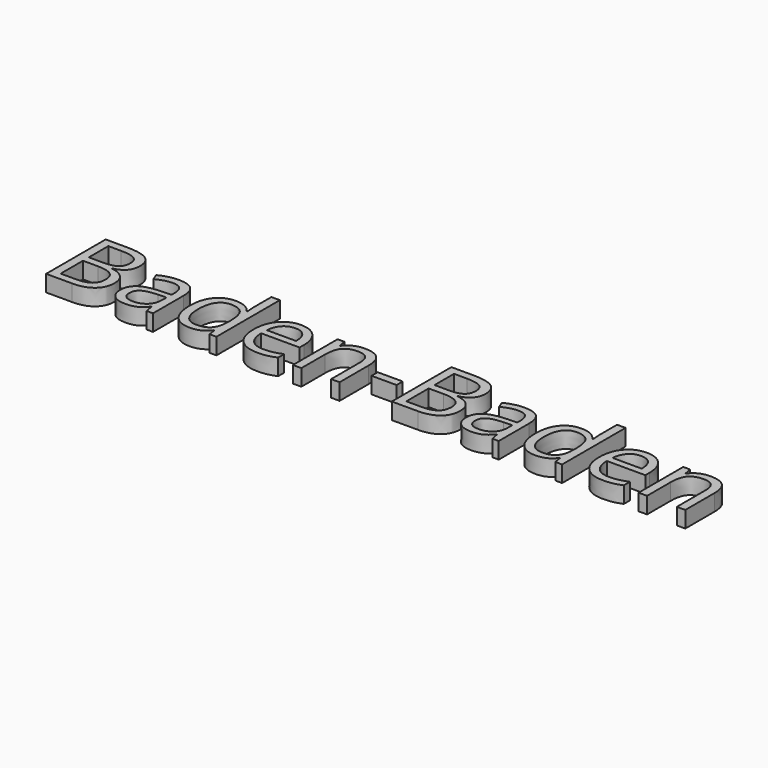
from build123d import *

# Parameters (mm, degrees)
F0_TEXT_SIZE = 12.7195488535
F1_DEPTH     = 2


# Not quite as in the source:
# - Text() gives the source's letters only with a copy of the font that has no kerning and outlines rounded to 1/6400 em; it was checked with that copy


with BuildPart() as f1:
    # F0 (on Top) → F1 (new body)
    with BuildSketch(Plane.XY):
        with Locations((-15.7074941643, -7.7180144344)):
            Text('Baden-Baden', F0_TEXT_SIZE, font='Open Sans', text_align=(TextAlign.LEFT, TextAlign.BOTTOM))
    extrude(amount=F1_DEPTH)


solid = f1.part
